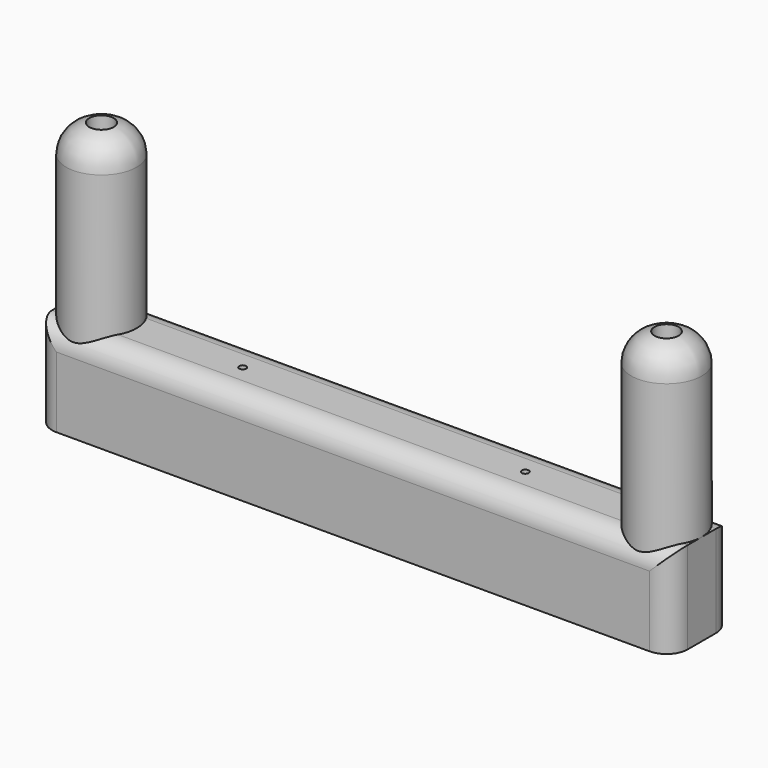
from build123d import *

# Parameters (mm, degrees)
F0_W         = 90
F0_H         = 11
F0_R         = 1.725
F0_R_2       = 1.7
F1_DEPTH     = 13
F2_R         = 5
F2_R_2       = 1.7
F3_DEPTH     = 24
F4_R         = 1.725
F5_DEPTH     = 24
F6_R         = 0.5
F7_DEPTH     = 12
F8_T1_DEPTH  = 28
F8_T6_DEPTH  = 105
F8_S7_R      = 5
F8_T8_DEPTH  = 54
F8_S9_R      = 5
F8_T10_DEPTH = 54
F8_T14_DEPTH = 105
F8_S15_R     = 5
F8_T16_DEPTH = 54
F8_S17_R     = 5
F8_T18_DEPTH = 54


# Not quite as in the source:
# - a fillet or chamfer that OpenCascade refuses, or shapes differently, is made with other operations: its cross-section is extruded or revolved along the edge and cut away or added
# - a feature names something its author has since deleted; it is built from what else it names


with BuildPart() as f1:
    # F0 (on Top) → F1 (new body)
    with BuildSketch(Plane.XY):
        Rectangle(F0_W, F0_H)
        with Locations((-40, 0)):
            Circle(F0_R, mode=Mode.SUBTRACT)
        with Locations((40, 0)):
            Circle(F0_R_2, mode=Mode.SUBTRACT)
    extrude(amount=F1_DEPTH)

    # F2 (on face) → F3 (join)
    with BuildSketch(Plane.XY.offset(13)):
        with Locations((40, 0)):
            Circle(F2_R)
        with Locations((40, 0)):
            Circle(F2_R_2, mode=Mode.SUBTRACT)
    extrude(amount=F3_DEPTH)

    # F4 (on face) → F5 (join)
    with BuildSketch(Plane.XY.offset(13)):
        with BuildLine():
            ThreePointArc((-45, 0), (-40, -5), (-35, 0))
            ThreePointArc((-35, 0), (-40, 5), (-45, 0))
        make_face()
        with Locations((-40, 0)):
            Circle(F4_R, mode=Mode.SUBTRACT)
    extrude(amount=F5_DEPTH)

    # F6 (on face) → F7 (cut)
    with BuildSketch(Plane.XY.offset(13)):
        with Locations((-20, 0)):
            Circle(F6_R)
        with Locations((20, 0)):
            Circle(F6_R)
    extrude(amount=-F7_DEPTH, mode=Mode.SUBTRACT)

    # F8: fillet of radius 3 on 6 edges, made by hand

    # F8_s2 → F8_t1 (cut)
    with BuildSketch(Plane.XY.offset(-7.5)):
        with BuildLine():
            ThreePointArc((-42, -5.5), (-44.1213203436, -4.6213203436), (-45, -2.5))
            Line((-45, -2.5), (-45, -5.5))
            Line((-45, -5.5), (-42, -5.5))
        make_face()
        with BuildLine():
            ThreePointArc((-45, 2.5), (-44.1213203436, 4.6213203436), (-42, 5.5))
            Line((-42, 5.5), (-45, 5.5))
            Line((-45, 5.5), (-45, 2.5))
        make_face()
        with BuildLine():
            ThreePointArc((42, -5.5), (44.1213203436, -4.6213203436), (45, -2.5))
            Line((45, -2.5), (45, -5.5))
            Line((45, -5.5), (42, -5.5))
        make_face()
        with BuildLine():
            ThreePointArc((45, 2.5), (44.1213203436, 4.6213203436), (42, 5.5))
            Line((42, 5.5), (45, 5.5))
            Line((45, 5.5), (45, 2.5))
        make_face()
    extrude(amount=F8_T1_DEPTH, mode=Mode.SUBTRACT)


with BuildPart() as f8_tool4:
    # F8_s5 → F8_t6 (new body)
    with BuildSketch(Plane.YZ.offset(-52.5)):
        with BuildLine():
            ThreePointArc((-5.5, 10), (-4.6213203436, 12.1213203436), (-2.5, 13))
            Line((-2.5, 13), (-5.5, 13))
            Line((-5.5, 13), (-5.5, 10))
        make_face()
    extrude(amount=F8_T6_DEPTH)

    # F8_s7 → F8_t8 (cut, symmetric)
    with BuildSketch(Plane.XY.offset(11.5)):
        with Locations((-40, 0)):
            Circle(F8_S7_R)
    extrude(amount=F8_T8_DEPTH, both=True, mode=Mode.SUBTRACT)

    # F8_s9 → F8_t10 (cut, symmetric)
    with BuildSketch(Plane.XY.offset(11.5)):
        with Locations((40, 0)):
            Circle(F8_S9_R)
    extrude(amount=F8_T10_DEPTH, both=True, mode=Mode.SUBTRACT)


with BuildPart() as f1_1:
    add(f1.part)

    # F8_t3: cut F8_tool4
    add(f8_tool4.part, mode=Mode.SUBTRACT)


with BuildPart() as f8_tool12:
    # F8_s13 → F8_t14 (new body)
    with BuildSketch(Plane.YZ.offset(52.5)):
        with BuildLine():
            ThreePointArc((2.5, 13), (4.6213203436, 12.1213203436), (5.5, 10))
            Line((5.5, 10), (5.5, 13))
            Line((5.5, 13), (2.5, 13))
        make_face()
    extrude(amount=-F8_T14_DEPTH)

    # F8_s15 → F8_t16 (cut, symmetric)
    with BuildSketch(Plane.XY.offset(11.5)):
        with Locations((-40, 0)):
            Circle(F8_S15_R)
    extrude(amount=F8_T16_DEPTH, both=True, mode=Mode.SUBTRACT)

    # F8_s17 → F8_t18 (cut, symmetric)
    with BuildSketch(Plane.XY.offset(11.5)):
        with Locations((40, 0)):
            Circle(F8_S17_R)
    extrude(amount=F8_T18_DEPTH, both=True, mode=Mode.SUBTRACT)


with BuildPart() as f1_2:
    add(f1_1.part)

    # F8_t11: cut F8_tool12
    add(f8_tool12.part, mode=Mode.SUBTRACT)

    # F9: fillet of radius 4 on 2 edges, made by hand

    # F9_s1 → F9_t2 (revolve, cut)
    with BuildSketch(Plane.XZ):
        with BuildLine():
            ThreePointArc((-38.275, 37), (-35.9259147702, 35.6255485658), (-35, 33.0662517874))
            Line((-35, 33.0662517874), (-35, 37))
            Line((-35, 37), (-38.275, 37))
        make_face()
    revolve(axis=Axis((-40, 0, 37), (0, 0, -1)), mode=Mode.SUBTRACT)

    # F9_s3 → F9_t4 (revolve, cut)
    with BuildSketch(Plane.XZ):
        with BuildLine():
            ThreePointArc((41.7, 37), (44.0659419434, 35.6307727822), (45, 33.0617262665))
            Line((45, 33.0617262665), (45, 37))
            Line((45, 37), (41.7, 37))
        make_face()
    revolve(axis=Axis((40, 0, 37), (0, 0, 1)), mode=Mode.SUBTRACT)


solid = f1_2.part
